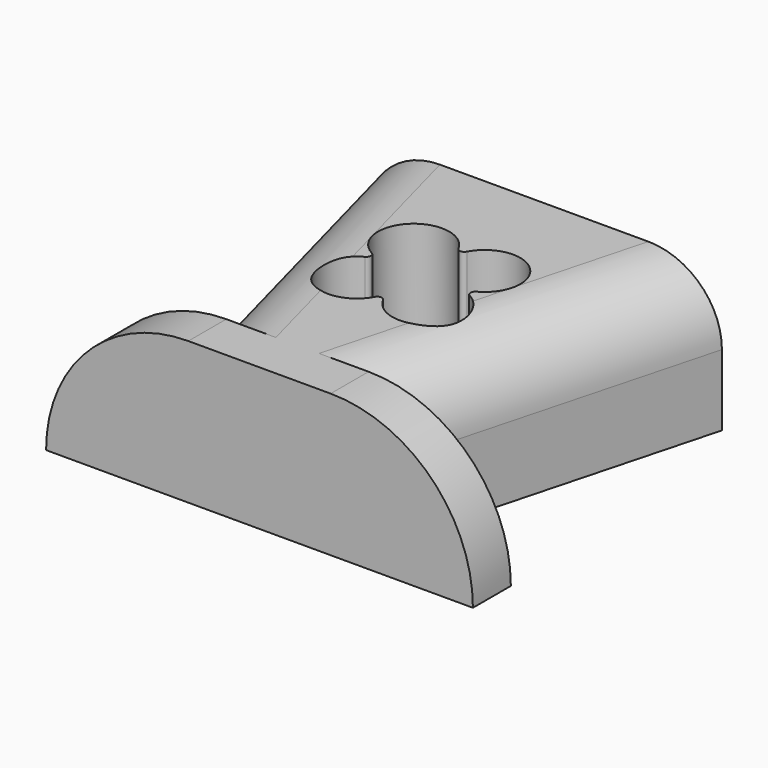
from build123d import *

# Parameters (mm, degrees)
F1_DEPTH    = 6
F2_F1_R     = 0.2
F2_F2_R     = 0.2
F3_T4_DEPTH = 28.4585903453
F3_T9_DEPTH = 28.4585903453
F4_R        = 5.99999


# Not quite as in the source:
# - a fillet or chamfer that OpenCascade refuses, or shapes differently, is made with other operations: its cross-section is extruded or revolved along the edge and cut away or added
# - a fillet or chamfer is up to 0.001 mm smaller than in the source, because OpenCascade refuses the exact size


with BuildPart() as f1:
    # F0 (on Top) → F1 (new body)
    with BuildSketch(Plane.XY):
        Polygon((-7.5, 8), (-4.418584287, -3.5), (4.418584287, -3.5), (7.5, 8), align=None)
        with BuildLine():
            ThreePointArc((-1.5, 1.5), (-2.5606601718, 4.0606601718), (0, 3))
            ThreePointArc((0, 3), (2.5606601718, 4.0606601718), (1.5, 1.5))
            ThreePointArc((1.5, 1.5), (2.5606601718, -1.0606601718), (0, 0))
            ThreePointArc((0, 0), (-2.5606601718, -1.0606601718), (-1.5, 1.5))
        make_face(mode=Mode.SUBTRACT)
        Polygon((-9, -5), (-9, -7), (9, -7), (9, -5), (4.0166604984, -5), (-4.0166604984, -5), align=None)
        Polygon((-4.418584287, -3.5), (-4.0166604984, -5), (4.0166604984, -5), (4.418584287, -3.5), align=None)
    extrude(amount=F1_DEPTH)

    # F2: fillet of radius 0.2 on 4 edges, made by hand

    # F2_f1
    f2_f1_edges = [f1.edges().sort_by_distance(p)[0] for p in [
        (-1.5, 1.5, 3),
        (0, 3, 3),
        (1.5, 1.5, 3),
    ]]
    fillet(f2_f1_edges, radius=F2_F1_R)

    # F2_f2
    f2_f2_edges = [f1.edges().sort_by_distance(p)[0] for p in [
        (0, 0, 3),
    ]]
    fillet(f2_f2_edges, radius=F2_F2_R)

    # F3: fillet of radius 3 on 2 edges, made by hand


with BuildPart() as f3_tool2:
    # F3_s3 → F3_t4 (new body)
    with BuildSketch(Plane(origin=(-4.4435475741, 16.5835453123, 0), x_dir=(0, 0, 1), z_dir=(0.2588190451, -0.9659258263, 0))):
        with BuildLine():
            ThreePointArc((3, 5.1738913363), (5.1213203436, 4.2952116799), (6, 2.1738913363))
            Line((6, 2.1738913363), (6, 5.1738913363))
            Line((6, 5.1738913363), (3, 5.1738913363))
        make_face()
    extrude(amount=F3_T4_DEPTH)

    split(bisect_by=Plane.XZ.offset(5), keep=Keep.BOTTOM)


with BuildPart() as f1_1:
    add(f1.part)

    # F3_t1: cut F3_tool2
    add(f3_tool2.part, mode=Mode.SUBTRACT)


with BuildPart() as f3_tool7:
    # F3_s8 → F3_t9 (new body)
    with BuildSketch(Plane(origin=(-2.9220776041, -10.905342082, 0), x_dir=(0, 0, 1), z_dir=(0.2588190451, 0.9659258263, 0))):
        with BuildLine():
            ThreePointArc((3, 5.1738913363), (5.1213203436, 4.2952116799), (6, 2.1738913363))
            Line((6, 2.1738913363), (6, 5.1738913363))
            Line((6, 5.1738913363), (3, 5.1738913363))
        make_face()
    extrude(amount=F3_T9_DEPTH)

    split(bisect_by=Plane.XZ.offset(5), keep=Keep.BOTTOM)


with BuildPart() as f1_2:
    add(f1_1.part)

    # F3_t6: cut F3_tool7
    add(f3_tool7.part, mode=Mode.SUBTRACT)

    # F4 (radius 6 in the source; OpenCascade refuses exactly that, so slightly less here)
    f4_edges = [f1_2.edges().sort_by_distance(p)[0] for p in [
        (9, -6, 6),
        (-9, -6, 6),
    ]]
    fillet(f4_edges, radius=F4_R)


solid = f1_2.part
